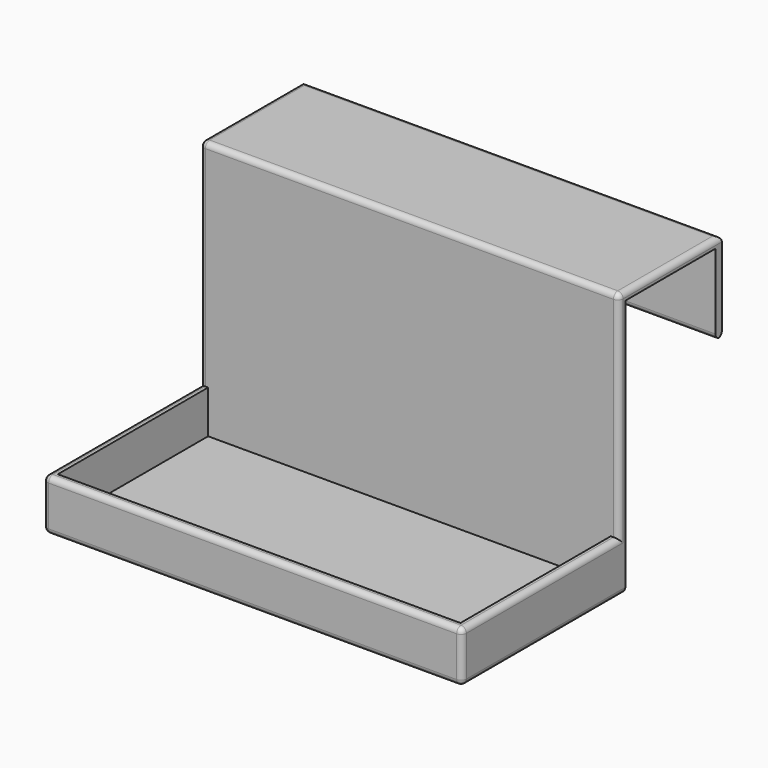
from build123d import *

# Parameters (mm, degrees)
F1_DEPTH     = 156
F2_W         = 150
F2_H         = 70
F3_DEPTH     = 16
F4_T1_DEPTH  = 152
F4_T3_DEPTH  = 51
F4_T5_DEPTH  = 166
F4_T7_DEPTH  = 78
F4_T9_DEPTH  = 71
F4_T11_DEPTH = 79
F4_T13_DEPTH = 15
F4_S17_W     = 2
F4_S17_H     = 2
F4_T18_DEPTH = 2
F4_S23_W     = 2
F4_S23_H     = 2
F4_T24_DEPTH = 2
F4_S29_W     = 2
F4_S29_H     = 2
F4_T30_DEPTH = 2
F4_S35_W     = 2
F4_S35_H     = 2
F4_T36_DEPTH = 2
F4_S41_W     = 2
F4_S41_H     = 2
F4_T42_DEPTH = 2
F4_S47_W     = 2
F4_S47_H     = 2
F4_T48_DEPTH = 2
F4_T55_DEPTH = 83
F4_T59_DEPTH = 76
F4_T66_DEPTH = 83
F4_T70_DEPTH = 76


# Not quite as in the source:
# - a fillet or chamfer that OpenCascade refuses, or shapes differently, is made with other operations: its cross-section is extruded or revolved along the edge and cut away or added


with BuildPart() as f1:
    # F0 (on Right) → F1 (new body)
    with BuildSketch(Plane.YZ):
        Polygon((3, -99), (3, -3), (0, -3), (0, -80), (-73, -80), (-73, -99), align=None)
        Polygon((0, -3), (3, -3), (45, -3), (45, 0), (0, 0), align=None)
        Polygon((45, 0), (45, -3), (45, -33), (48, -33), (48, 0), align=None)
    extrude(amount=F1_DEPTH)

    # F2 (on face) → F3 (cut)
    with BuildSketch(Plane.XY.offset(-80)):
        with Locations((78, -35)):
            Rectangle(F2_W, F2_H)
    extrude(amount=-F3_DEPTH, mode=Mode.SUBTRACT)

    # F4: fillet of radius 2 on 16 edges, made by hand

    # F4_s2 → F4_t1 (cut)
    with BuildSketch(Plane.YZ.offset(2)):
        with BuildLine():
            ThreePointArc((2, 0), (0.5857864376, -0.5857864376), (0, -2))
            Line((0, -2), (0, 0))
            Line((0, 0), (2, 0))
        make_face()
        with BuildLine():
            ThreePointArc((-73, -82), (-72.4142135624, -80.5857864376), (-71, -80))
            Line((-71, -80), (-73, -80))
            Line((-73, -80), (-73, -82))
        make_face()
        with BuildLine():
            ThreePointArc((-71, -99), (-72.4142135624, -98.4142135624), (-73, -97))
            Line((-73, -97), (-73, -99))
            Line((-73, -99), (-71, -99))
        make_face()
    extrude(amount=F4_T1_DEPTH, mode=Mode.SUBTRACT)

    # F4_s4 → F4_t3 (cut)
    with BuildSketch(Plane.XZ.offset(-53)):
        with BuildLine():
            ThreePointArc((156, -2), (155.4142135624, -0.5857864376), (154, 0))
            Line((154, 0), (156, 0))
            Line((156, 0), (156, -2))
        make_face()
        with BuildLine():
            ThreePointArc((0, -2), (0.5857864376, -0.5857864376), (2, 0))
            Line((2, 0), (0, 0))
            Line((0, 0), (0, -2))
        make_face()
    extrude(amount=F4_T3_DEPTH, mode=Mode.SUBTRACT)

    # F4_s6 → F4_t5 (cut)
    with BuildSketch(Plane.YZ.offset(-5)):
        with BuildLine():
            ThreePointArc((48, -2), (47.4142135624, -0.5857864376), (46, 0))
            Line((46, 0), (48, 0))
            Line((48, 0), (48, -2))
        make_face()
        with BuildLine():
            ThreePointArc((46, -33), (47.4142135624, -32.4142135624), (48, -31))
            Line((48, -31), (48, -33))
            Line((48, -33), (46, -33))
        make_face()
        with BuildLine():
            ThreePointArc((45, -31), (45.5857864376, -32.4142135624), (47, -33))
            Line((47, -33), (45, -33))
            Line((45, -33), (45, -31))
        make_face()
    extrude(amount=F4_T5_DEPTH, mode=Mode.SUBTRACT)

    # F4_s8 → F4_t7 (cut)
    with BuildSketch(Plane.XY.offset(-80)):
        with BuildLine():
            ThreePointArc((156, 2), (155.4142135624, 0.5857864376), (154, 0))
            Line((154, 0), (156, 0))
            Line((156, 0), (156, 2))
        make_face()
        with BuildLine():
            ThreePointArc((0, 2), (0.5857864376, 0.5857864376), (2, 0))
            Line((2, 0), (0, 0))
            Line((0, 0), (0, 2))
        make_face()
    extrude(amount=F4_T7_DEPTH, mode=Mode.SUBTRACT)

    # F4_s10 → F4_t9 (cut)
    with BuildSketch(Plane.XZ):
        with BuildLine():
            ThreePointArc((156, -82), (155.4142135624, -80.5857864376), (154, -80))
            Line((154, -80), (156, -80))
            Line((156, -80), (156, -82))
        make_face()
        with BuildLine():
            ThreePointArc((0, -82), (0.5857864376, -80.5857864376), (2, -80))
            Line((2, -80), (0, -80))
            Line((0, -80), (0, -82))
        make_face()
    extrude(amount=F4_T9_DEPTH, mode=Mode.SUBTRACT)

    # F4_s12 → F4_t11 (cut)
    with BuildSketch(Plane.XZ.offset(-8)):
        with BuildLine():
            ThreePointArc((154, -99), (155.4142135624, -98.4142135624), (156, -97))
            Line((156, -97), (156, -99))
            Line((156, -99), (154, -99))
        make_face()
        with BuildLine():
            ThreePointArc((2, -99), (0.5857864376, -98.4142135624), (0, -97))
            Line((0, -97), (0, -99))
            Line((0, -99), (2, -99))
        make_face()
    extrude(amount=F4_T11_DEPTH, mode=Mode.SUBTRACT)

    # F4_s14 → F4_t13 (cut)
    with BuildSketch(Plane.XY.offset(-97)):
        with BuildLine():
            ThreePointArc((0, -71), (0.5857864376, -72.4142135624), (2, -73))
            Line((2, -73), (0, -73))
            Line((0, -73), (0, -71))
        make_face()
        with BuildLine():
            ThreePointArc((156, -71), (155.4142135624, -72.4142135624), (154, -73))
            Line((154, -73), (156, -73))
            Line((156, -73), (156, -71))
        make_face()
    extrude(amount=F4_T13_DEPTH, mode=Mode.SUBTRACT)


with BuildPart() as f4_tool16:
    # F4_s17 → F4_t18 (new body)
    with BuildSketch(Plane.XY.offset(-2)):
        with Locations((1, 1)):
            Rectangle(F4_S17_W, F4_S17_H)
    extrude(amount=F4_T18_DEPTH)

    # F4_s19 → F4_t20 (revolve, cut)
    with BuildSketch(Plane(origin=(2, 2, -2), x_dir=(0.7071067812, 0.7071067812, 0), z_dir=(0.7071067812, -0.7071067812, 0))):
        with BuildLine():
            ThreePointArc((0, -2), (2, 0), (0, 2))
            Line((0, 2), (0, -2))
        make_face()
    revolve(axis=Axis((2, 2, -2), (0, 0, 1)), mode=Mode.SUBTRACT)


with BuildPart() as f1_1:
    add(f1.part)

    # F4_t15: cut F4_tool16
    add(f4_tool16.part, mode=Mode.SUBTRACT)


with BuildPart() as f4_tool22:
    # F4_s23 → F4_t24 (new body)
    with BuildSketch(Plane.XY.offset(-2)):
        with Locations((155, 1)):
            Rectangle(F4_S23_W, F4_S23_H)
    extrude(amount=F4_T24_DEPTH)

    # F4_s25 → F4_t26 (revolve, cut)
    with BuildSketch(Plane(origin=(154, 2, -2), x_dir=(-0.7071067812, 0.7071067812, 0), z_dir=(0.7071067812, 0.7071067812, 0))):
        with BuildLine():
            ThreePointArc((0, -2), (2, 0), (0, 2))
            Line((0, 2), (0, -2))
        make_face()
    revolve(axis=Axis((154, 2, -2), (0, 0, 1)), mode=Mode.SUBTRACT)


with BuildPart() as f1_2:
    add(f1_1.part)

    # F4_t21: cut F4_tool22
    add(f4_tool22.part, mode=Mode.SUBTRACT)


with BuildPart() as f4_tool28:
    # F4_s29 → F4_t30 (new body)
    with BuildSketch(Plane.XY.offset(-82)):
        with Locations((155, -72)):
            Rectangle(F4_S29_W, F4_S29_H)
    extrude(amount=F4_T30_DEPTH)

    # F4_s31 → F4_t32 (revolve, cut)
    with BuildSketch(Plane(origin=(154, -71, -82), x_dir=(-0.7071067812, 0.7071067812, 0), z_dir=(0.7071067812, 0.7071067812, 0))):
        with BuildLine():
            ThreePointArc((0, -2), (2, 0), (0, 2))
            Line((0, 2), (0, -2))
        make_face()
    revolve(axis=Axis((154, -71, -82), (0, 0, 1)), mode=Mode.SUBTRACT)


with BuildPart() as f1_3:
    add(f1_2.part)

    # F4_t27: cut F4_tool28
    add(f4_tool28.part, mode=Mode.SUBTRACT)


with BuildPart() as f4_tool34:
    # F4_s35 → F4_t36 (new body)
    with BuildSketch(Plane.YZ.offset(2)):
        with Locations((-72, -81)):
            Rectangle(F4_S35_W, F4_S35_H)
    extrude(amount=-F4_T36_DEPTH)

    # F4_s37 → F4_t38 (revolve, cut)
    with BuildSketch(Plane(origin=(2, -71, -82), x_dir=(0, 0.7071067812, -0.7071067812), z_dir=(0, 0.7071067812, 0.7071067812))):
        with BuildLine():
            ThreePointArc((0, -2), (2, 0), (0, 2))
            Line((0, 2), (0, -2))
        make_face()
    revolve(axis=Axis((2, -71, -82), (-1, 0, 0)), mode=Mode.SUBTRACT)


with BuildPart() as f1_4:
    add(f1_3.part)

    # F4_t33: cut F4_tool34
    add(f4_tool34.part, mode=Mode.SUBTRACT)


with BuildPart() as f4_tool40:
    # F4_s41 → F4_t42 (new body)
    with BuildSketch(Plane.XY.offset(-97)):
        with Locations((1, -72)):
            Rectangle(F4_S41_W, F4_S41_H)
    extrude(amount=-F4_T42_DEPTH)

    # F4_s43 → F4_t44 (revolve, cut)
    with BuildSketch(Plane(origin=(2, -71, -97), x_dir=(0.7071067812, 0.7071067812, 0), z_dir=(-0.7071067812, 0.7071067812, 0))):
        with BuildLine():
            ThreePointArc((0, -2), (2, 0), (0, 2))
            Line((0, 2), (0, -2))
        make_face()
    revolve(axis=Axis((2, -71, -97), (0, 0, -1)), mode=Mode.SUBTRACT)


with BuildPart() as f1_5:
    add(f1_4.part)

    # F4_t39: cut F4_tool40
    add(f4_tool40.part, mode=Mode.SUBTRACT)


with BuildPart() as f4_tool46:
    # F4_s47 → F4_t48 (new body)
    with BuildSketch(Plane.XY.offset(-97)):
        with Locations((155, -72)):
            Rectangle(F4_S47_W, F4_S47_H)
    extrude(amount=-F4_T48_DEPTH)

    # F4_s49 → F4_t50 (revolve, cut)
    with BuildSketch(Plane(origin=(154, -71, -97), x_dir=(-0.7071067812, 0.7071067812, 0), z_dir=(-0.7071067812, -0.7071067812, 0))):
        with BuildLine():
            ThreePointArc((0, -2), (2, 0), (0, 2))
            Line((0, 2), (0, -2))
        make_face()
    revolve(axis=Axis((154, -71, -97), (0, 0, -1)), mode=Mode.SUBTRACT)


with BuildPart() as f1_6:
    add(f1_5.part)

    # F4_t45: cut F4_tool46
    add(f4_tool46.part, mode=Mode.SUBTRACT)


with BuildPart() as f4_tool53:
    # F4_s54 → F4_t55 (new body)
    with BuildSketch(Plane.XY.offset(-2)):
        with BuildLine():
            ThreePointArc((156, 2), (155.4142135624, 0.5857864376), (154, 0))
            Line((154, 0), (156, 0))
            Line((156, 0), (156, 2))
        make_face()
    extrude(amount=-F4_T55_DEPTH)

    split(bisect_by=Plane.XY.offset(-80), keep=Keep.BOTTOM)


with BuildPart() as f4_tool57:
    # F4_s58 → F4_t59 (new body)
    with BuildSketch(Plane.XZ.offset(-5)):
        with BuildLine():
            ThreePointArc((156, -82), (155.4142135624, -80.5857864376), (154, -80))
            Line((154, -80), (156, -80))
            Line((156, -80), (156, -82))
        make_face()
    extrude(amount=F4_T59_DEPTH)

    split(bisect_by=Plane.XZ, keep=Keep.BOTTOM)


with BuildPart() as f4_tool53_1:
    add(f4_tool53.part)

    # F4_t61: intersect F4_tool57
    add(f4_tool57.part, mode=Mode.INTERSECT)


with BuildPart() as f1_7:
    add(f1_6.part)

    # F4_t51: cut F4_tool53
    add(f4_tool53_1.part, mode=Mode.SUBTRACT)


with BuildPart() as f4_tool64:
    # F4_s65 → F4_t66 (new body)
    with BuildSketch(Plane.XY.offset(-2)):
        with BuildLine():
            ThreePointArc((0, 2), (0.5857864376, 0.5857864376), (2, 0))
            Line((2, 0), (0, 0))
            Line((0, 0), (0, 2))
        make_face()
    extrude(amount=-F4_T66_DEPTH)

    split(bisect_by=Plane.XY.offset(-80), keep=Keep.BOTTOM)


with BuildPart() as f4_tool68:
    # F4_s69 → F4_t70 (new body)
    with BuildSketch(Plane.XZ.offset(-5)):
        with BuildLine():
            ThreePointArc((0, -82), (0.5857864376, -80.5857864376), (2, -80))
            Line((2, -80), (0, -80))
            Line((0, -80), (0, -82))
        make_face()
    extrude(amount=F4_T70_DEPTH)

    split(bisect_by=Plane.XZ, keep=Keep.BOTTOM)


with BuildPart() as f4_tool64_1:
    add(f4_tool64.part)

    # F4_t72: intersect F4_tool68
    add(f4_tool68.part, mode=Mode.INTERSECT)


with BuildPart() as f1_8:
    add(f1_7.part)

    # F4_t62: cut F4_tool64
    add(f4_tool64_1.part, mode=Mode.SUBTRACT)


solid = f1_8.part
